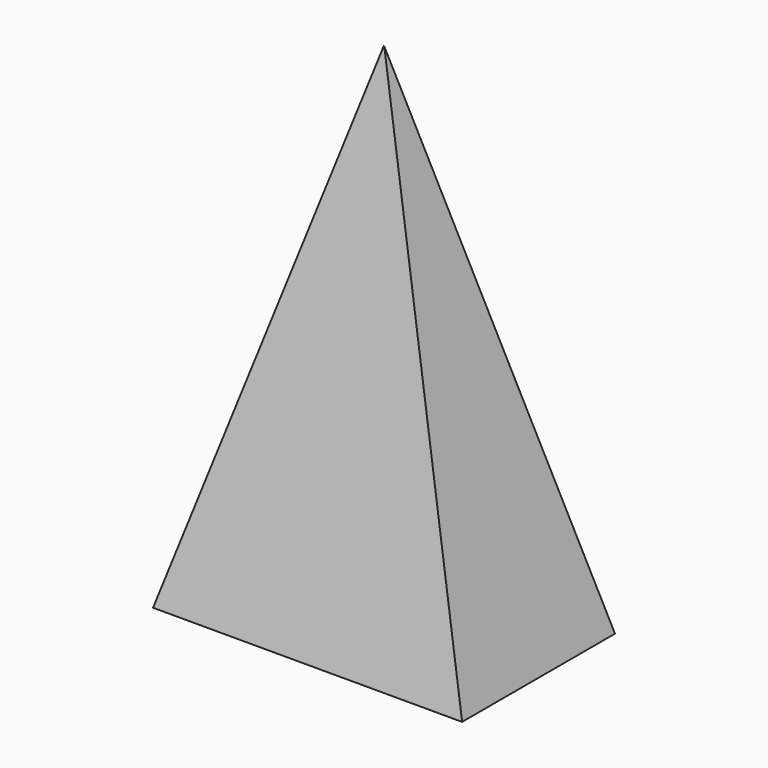
from build123d import *

# Parameters (mm, degrees)
F0_W       = 139.7
F0_H       = 86.36
F1_DEPTH   = 228.6
F2_SIZE2   = 69.72299
F2_SIZE    = 228.59999
F2_2_SIZE2 = 69.72299
F2_2_SIZE  = 228.59999
F3_SIZE2   = 228.59999
F3_SIZE    = 43.17999


# Not quite as in the source:
# - a fillet or chamfer is up to 0.001 mm smaller than in the source, because OpenCascade refuses the exact size


with BuildPart() as f1:
    # F0 (on Top) → F1 (new body)
    with BuildSketch(Plane.XY):
        Rectangle(F0_W, F0_H)
    extrude(amount=F1_DEPTH)

    # F2 (size 228.6 and 69.723 in the source; OpenCascade refuses exactly that, so slightly less here)
    f2_edges = [f1.edges().sort_by_distance(p)[0] for p in [
        (69.85, 0, 228.6),
    ]]
    f2_side = f1.faces().sort_by_distance((69.85, 0, 114.3))[0]
    chamfer(f2_edges, length=F2_SIZE, length2=F2_SIZE2, reference=f2_side)

    # F2#2 (size 228.6 and 69.723 in the source; OpenCascade refuses exactly that, so slightly less here)
    f2_2_edges = [f1.edges().sort_by_distance(p)[0] for p in [
        (-69.85, 0, 228.6),
    ]]
    f2_2_side = f1.faces().sort_by_distance((-69.85, 0, 114.3))[0]
    chamfer(f2_2_edges, length=F2_2_SIZE, length2=F2_2_SIZE2, reference=f2_2_side)

    # F3 (size 43.18 and 228.6 in the source; OpenCascade refuses exactly that, so slightly less here)
    f3_edges = [f1.edges().sort_by_distance(p)[0] for p in [
        (0, -43.18, 228.6),
        (0, 43.18, 228.6),
    ]]
    f3_side = f1.faces().sort_by_distance((0, 0, 228.6))[0]
    chamfer(f3_edges, length=F3_SIZE, length2=F3_SIZE2, reference=f3_side)


solid = f1.part
